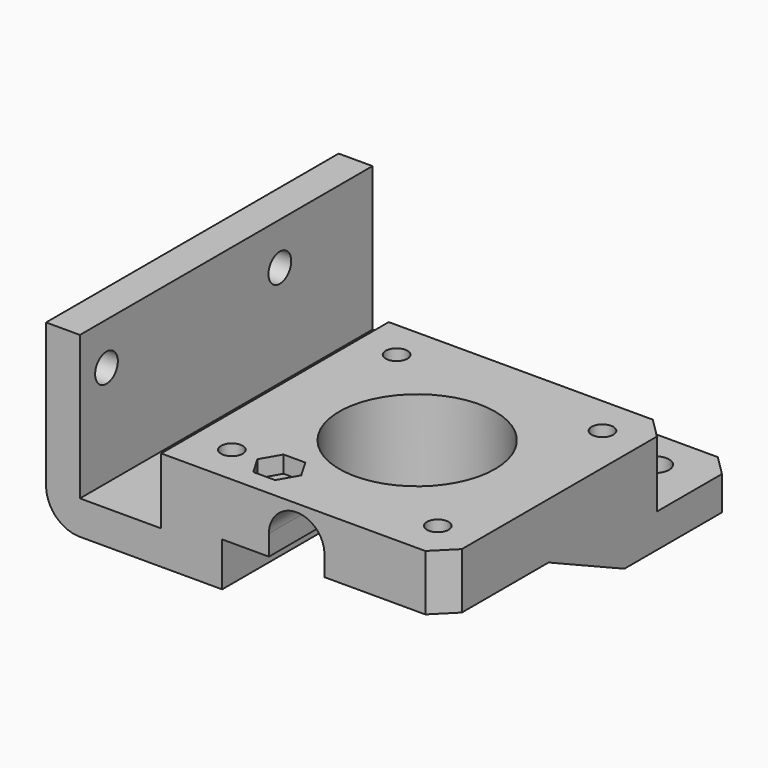
from build123d import *

# Parameters (mm, degrees)
F0_W      = 59
F0_H      = 54
F1_DEPTH  = 5
F2_W      = 5
F2_H      = 54
F3_DEPTH  = 21.25
F4_W      = 42
F4_H      = 42
F5_DEPTH  = 9.75
F7_DEPTH  = 33
F8_R      = 1.6
F8_R_2    = 11.5
F9_DEPTH  = 14.751
F10_R     = 2.1
F11_DEPTH = 5.001
F12_SIZE  = 3
F13_R     = 5
F14_R     = 1.6
F15_DEPTH = 2.5
F16_R     = 2.1
F17_DEPTH = 59.001
F19_DEPTH = 10.6937211186


with BuildPart() as f1:
    # F0 (on Top) → F1 (new body)
    with BuildSketch(Plane.XY):
        with Locations((29.5, 27)):
            Rectangle(F0_W, F0_H)
    extrude(amount=F1_DEPTH)

    # F2 (on face) → F3 (join)
    with BuildSketch(Plane.XY.offset(5)):
        with Locations((2.5, 27)):
            Rectangle(F2_W, F2_H)
    extrude(amount=F3_DEPTH)

    # F4 (on face) → F5 (join)
    with BuildSketch(Plane.XY.offset(5)):
        with Locations((38, 21)):
            Rectangle(F4_W, F4_H)
    extrude(amount=F5_DEPTH)

    # F6 (on face) → F7 (cut)
    with BuildSketch(Plane.YZ.offset(59)):
        Polygon((0, 6.5), (0, 0), (33, 0), (19, 6.5), align=None)
    extrude(amount=-F7_DEPTH, mode=Mode.SUBTRACT)

    # F8 (on face) → F9 (cut, through all)
    with BuildSketch(Plane.XY.offset(14.75)):
        with Locations((22.8, 36.2)):
            Circle(F8_R)
        with Locations((38, 21)):
            Circle(F8_R_2)
        with Locations((53.2, 36.2)):
            Circle(F8_R)
        with Locations((22.8, 5.8)):
            Circle(F8_R)
        with Locations((53.2, 5.8)):
            Circle(F8_R)
        with Locations((29.8, 5.8)):
            Circle(F8_R)
    extrude(amount=-F9_DEPTH, mode=Mode.SUBTRACT)

    # F10 (on face) → F11 (cut, through all)
    with BuildSketch(Plane.XY.offset(5)):
        with Locations((37, 48)):
            Circle(F10_R)
        with Locations((51.5, 48)):
            Circle(F10_R)
    extrude(amount=-F11_DEPTH, mode=Mode.SUBTRACT)

    # F12
    f12_edges = [f1.edges().sort_by_distance(p)[0] for p in [
        (59, 54, 2.5),
        (59, 42, 9.875),
        (59, 0, 10.625),
    ]]
    chamfer(f12_edges, length=F12_SIZE)

    # F13
    f13_edges = [f1.edges().sort_by_distance(p)[0] for p in [
        (0, 27, 0),
    ]]
    fillet(f13_edges, radius=F13_R)

    # F14 (on face) → F15 (cut)
    with BuildSketch(Plane.XY.offset(14.75)):
        Polygon((31.417729554, 3.0006632601), (33.0331615075, 5.8013265202), (31.4154319535, 8.6006632601), (28.182270446, 8.5993367399), (26.5668384925, 5.7986734798), (28.1845680465, 2.9993367399), align=None)
        with Locations((29.8, 5.8)):
            Circle(F14_R, mode=Mode.SUBTRACT)
    extrude(amount=-F15_DEPTH, mode=Mode.SUBTRACT)

    # F16 (on face) → F17 (cut, through all)
    with BuildSketch(Plane(origin=(0, 0, 0), x_dir=(0, -1, 0), z_dir=(-1, 0, 0))):
        with Locations((-36.9, 20)):
            Circle(F16_R)
        with Locations((-4.9, 20)):
            Circle(F16_R)
    extrude(amount=-F17_DEPTH, mode=Mode.SUBTRACT)

    # F18 (on face) → F19 (cut, through all)
    with BuildSketch(Plane.XZ):
        with BuildLine():
            Line((32.9, 9.5), (32.9, 6.5))
            Line((32.9, 6.5), (41.1, 6.5))
            Line((41.1, 6.5), (41.1, 9.5))
            ThreePointArc((41.1, 9.5), (37, 13.6), (32.9, 9.5))
        make_face()
    extrude(amount=-F19_DEPTH, mode=Mode.SUBTRACT)


solid = f1.part
